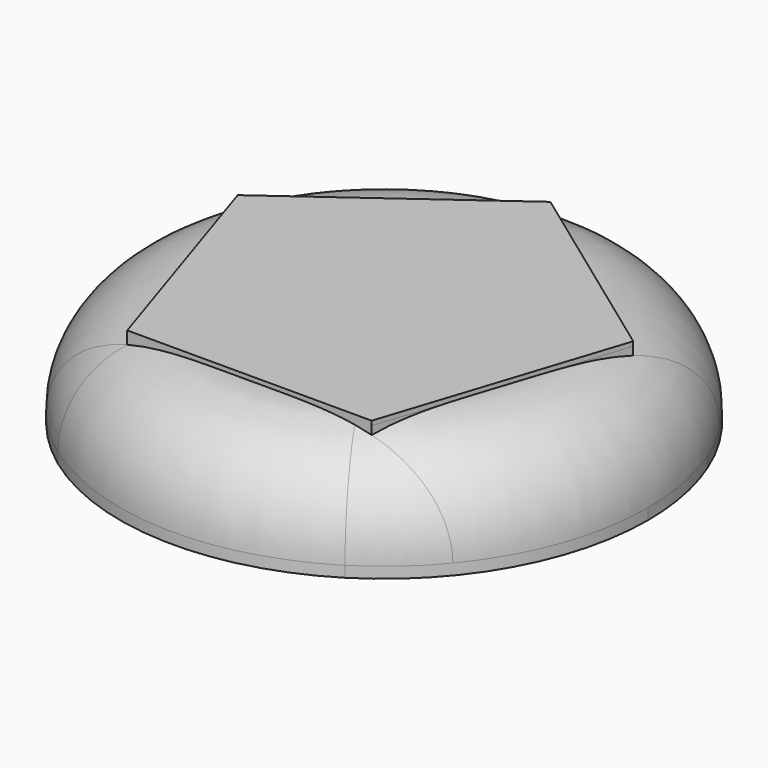
from build123d import *

# Parameters (mm, degrees)
F1_DEPTH     = 12.7
F2_DEPTH     = 12.192
F3_DEPTH     = 12.192
F4_DEPTH     = 12.192
F5_DEPTH     = 12.192
F6_DEPTH     = 12.192
F7_T4_ANGLE  = 291.9758344639
F7_T9_ANGLE  = 291.9758344639
F7_T14_ANGLE = 291.9758344639
F7_T19_ANGLE = 291.9758344639
F7_T24_ANGLE = 291.9758344639
F7_T29_ANGLE = 68.0241655361


# Not quite as in the source:
# - a fillet or chamfer that OpenCascade refuses, or shapes differently, is made with other operations: its cross-section is extruded or revolved along the edge and cut away or added


with BuildPart() as f1:
    # F0 (on Top) → F1 (new body)
    with BuildSketch(Plane.XY):
        Polygon((0, 24.0160203306), (-22.8405926309, 7.4213584194), (-14.1162625691, -19.4293685847), (14.1162625691, -19.4293685847), (22.8405926309, 7.4213584194), align=None)
    extrude(amount=F1_DEPTH)

    # F0 (on Top) → F2 (join)
    with BuildSketch(Plane.XY):
        with BuildLine():
            Line((-14.1162625691, -19.4293685847), (-22.8405926309, 7.4213584194))
            Line((-22.8405926309, 7.4213584194), (-28.2653771262, 11.4060885458))
            ThreePointArc((-28.2653771262, 11.4060885458), (-29.2974841135, -8.4076051653), (-17.9156944899, -24.6588379885))
            Line((-17.9156944899, -24.6588379885), (-14.1162625691, -19.4293685847))
        make_face()
    extrude(amount=F2_DEPTH)

    # F0 (on Top) → F3 (join)
    with BuildSketch(Plane.XY):
        with BuildLine():
            Line((-28.2653771262, 11.4060885458), (-22.8405926309, 7.4213584194))
            Line((-22.8405926309, 7.4213584194), (0, 24.0160203306))
            Line((0, 24.0160203306), (0, 30.48))
            ThreePointArc((0, 30.48), (-17.0495281625, 25.2654702992), (-28.2653771262, 11.4060885458))
        make_face()
    extrude(amount=F3_DEPTH)

    # F0 (on Top) → F4 (join)
    with BuildSketch(Plane.XY):
        with BuildLine():
            Line((0, 30.48), (0, 24.0160203306))
            Line((0, 24.0160203306), (22.8405926309, 7.4213584194))
            Line((22.8405926309, 7.4213584194), (28.2789000487, 11.3725200388))
            ThreePointArc((28.2789000487, 11.3725200388), (17.0645244472, 25.2553440957), (0, 30.48))
        make_face()
    extrude(amount=F4_DEPTH)

    # F0 (on Top) → F5 (join)
    with BuildSketch(Plane.XY):
        with BuildLine():
            Line((28.2789000487, 11.3725200388), (22.8405926309, 7.4213584194))
            Line((22.8405926309, 7.4213584194), (14.1162625691, -19.4293685847))
            Line((14.1162625691, -19.4293685847), (16.162839814, -25.8416912981))
            ThreePointArc((16.162839814, -25.8416912981), (26.6615243144, -14.7713750624), (30.48, 0))
            ThreePointArc((30.48, 0), (29.9246660256, 5.7917841169), (28.2789000487, 11.3725200388))
        make_face()
    extrude(amount=F5_DEPTH)

    # F0 (on Top) → F6 (join)
    with BuildSketch(Plane.XY):
        with BuildLine():
            Line((14.1162625691, -19.4293685847), (-14.1162625691, -19.4293685847))
            Line((-14.1162625691, -19.4293685847), (-17.9156944899, -24.6588379885))
            ThreePointArc((-17.9156944899, -24.6588379885), (-1.0573128046, -30.4616560553), (16.162839814, -25.8416912981))
            Line((16.162839814, -25.8416912981), (14.1162625691, -19.4293685847))
        make_face()
    extrude(amount=F6_DEPTH)

    # F7: fillet of radius 10.922 on 2 edges, made by hand


with BuildPart() as f7_tool2:
    # F7_s3 → F7_t4 (revolve)
    with BuildSketch(Plane(origin=(0, 0, 0), x_dir=(0, 0, 1), z_dir=(-0.8478245177, -0.5302768968, 0))):
        with BuildLine():
            ThreePointArc((12.192, -19.558), (8.9930202641, -27.2810202641), (1.27, -30.48))
            Line((1.27, -30.48), (12.192, -30.48))
            Line((12.192, -30.48), (12.192, -19.558))
        make_face()
    revolve(axis=Axis((0, 0, 12.192), (0, 0, 1)), revolution_arc=F7_T4_ANGLE)

    split(bisect_by=Plane.XZ.offset(19.4293685847), keep=Keep.TOP)


with BuildPart() as f1_1:
    add(f1.part)

    # F7_t1: cut F7_tool2
    add(f7_tool2.part, mode=Mode.SUBTRACT)


with BuildPart() as f7_tool7:
    # F7_s8 → F7_t9 (revolve)
    with BuildSketch(Plane(origin=(0, 0, 0), x_dir=(0, 0, 1), z_dir=(-0.8478245177, -0.5302768968, 0))):
        with BuildLine():
            ThreePointArc((12.192, -19.558), (8.9930202641, -27.2810202641), (1.27, -30.48))
            Line((1.27, -30.48), (12.192, -30.48))
            Line((12.192, -30.48), (12.192, -19.558))
        make_face()
    revolve(axis=Axis((0, 0, 12.192), (0, 0, 1)), revolution_arc=F7_T9_ANGLE)

    split(bisect_by=Plane(origin=(18.4784276, -6.0040050827, 0), x_dir=(0, 0, 1), z_dir=(0.9510565163, -0.3090169944, 0)), keep=Keep.TOP)


with BuildPart() as f1_2:
    add(f1_1.part)

    # F7_t6: cut F7_tool7
    add(f7_tool7.part, mode=Mode.SUBTRACT)


with BuildPart() as f7_tool12:
    # F7_s13 → F7_t14 (revolve)
    with BuildSketch(Plane(origin=(0, 0, 0), x_dir=(0, 0, 1), z_dir=(-0.8478245177, -0.5302768968, 0))):
        with BuildLine():
            ThreePointArc((12.192, -19.558), (8.9930202641, -27.2810202641), (1.27, -30.48))
            Line((1.27, -30.48), (12.192, -30.48))
            Line((12.192, -30.48), (12.192, -19.558))
        make_face()
    revolve(axis=Axis((0, 0, 12.192), (0, 0, 1)), revolution_arc=F7_T14_ANGLE)

    split(bisect_by=Plane(origin=(11.4202963155, 15.718689375, 0), x_dir=(0, 0, 1), z_dir=(0.5877852523, 0.8090169944, 0)), keep=Keep.TOP)


with BuildPart() as f1_3:
    add(f1_2.part)

    # F7_t11: cut F7_tool12
    add(f7_tool12.part, mode=Mode.SUBTRACT)


with BuildPart() as f7_tool17:
    # F7_s18 → F7_t19 (revolve)
    with BuildSketch(Plane(origin=(0, 0, 0), x_dir=(0, 0, 1), z_dir=(-0.8478245177, -0.5302768968, 0))):
        with BuildLine():
            ThreePointArc((12.192, -19.558), (8.9930202641, -27.2810202641), (1.27, -30.48))
            Line((1.27, -30.48), (12.192, -30.48))
            Line((12.192, -30.48), (12.192, -19.558))
        make_face()
    revolve(axis=Axis((0, 0, 12.192), (0, 0, 1)), revolution_arc=F7_T19_ANGLE)

    split(bisect_by=Plane(origin=(-11.4202963155, 15.718689375, 0), x_dir=(0, 0, 1), z_dir=(-0.5877852523, 0.8090169944, 0)), keep=Keep.TOP)


with BuildPart() as f1_4:
    add(f1_3.part)

    # F7_t16: cut F7_tool17
    add(f7_tool17.part, mode=Mode.SUBTRACT)


with BuildPart() as f7_tool22:
    # F7_s23 → F7_t24 (revolve)
    with BuildSketch(Plane(origin=(0, 0, 0), x_dir=(0, 0, 1), z_dir=(-0.8478245177, -0.5302768968, 0))):
        with BuildLine():
            ThreePointArc((12.192, -19.558), (8.9930202641, -27.2810202641), (1.27, -30.48))
            Line((1.27, -30.48), (12.192, -30.48))
            Line((12.192, -30.48), (12.192, -19.558))
        make_face()
    revolve(axis=Axis((0, 0, 12.192), (0, 0, 1)), revolution_arc=F7_T24_ANGLE)

    split(bisect_by=Plane(origin=(-18.4784276, -6.0040050827, 0), x_dir=(0, 0, 1), z_dir=(-0.9510565163, -0.3090169944, 0)), keep=Keep.TOP)


with BuildPart() as f1_5:
    add(f1_4.part)

    # F7_t21: cut F7_tool22
    add(f7_tool22.part, mode=Mode.SUBTRACT)


with BuildPart() as f7_tool27:
    # F7_s28 → F7_t29 (revolve)
    with BuildSketch(Plane(origin=(0, 0, 0), x_dir=(0, 0, 1), z_dir=(-0.8090169944, 0.5877852523, 0))):
        with BuildLine():
            ThreePointArc((12.192, -19.558), (8.9930202641, -27.2810202641), (1.27, -30.48))
            Line((1.27, -30.48), (12.192, -30.48))
            Line((12.192, -30.48), (12.192, -19.558))
        make_face()
    revolve(axis=Axis((0, 0, 12.192), (0, 0, 1)), revolution_arc=F7_T29_ANGLE)

    split(bisect_by=Plane.XZ.offset(19.4293685847), keep=Keep.TOP)


with BuildPart() as f1_6:
    add(f1_5.part)

    # F7_t26: cut F7_tool27
    add(f7_tool27.part, mode=Mode.SUBTRACT)


solid = f1_6.part
